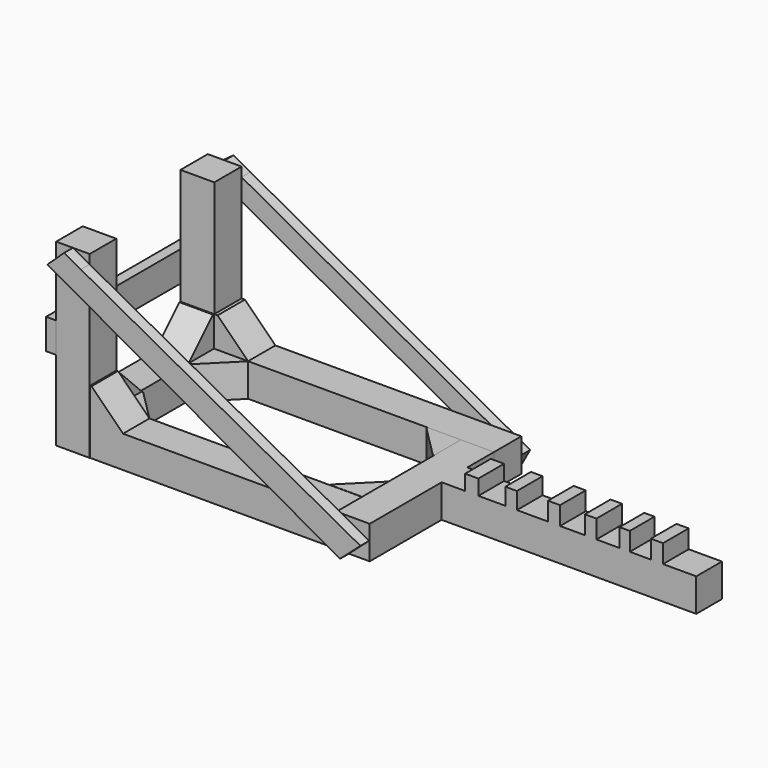
from build123d import *

# Parameters (mm, degrees)
F1_W         = 151.4005884528
F1_H         = 15.9740373492
F2_DEPTH     = 15.494
F3_W         = 151.6942754388
F3_H         = 16.5184233338
F4_DEPTH     = 16.002
F5_W         = 16.2231996655
F5_H         = 16.002
F6_DEPTH     = 75.184
F7_W         = 16.0225182772
F7_H         = 16.002
F8_DEPTH     = 75.184
F9_W         = 16.3512788713
F9_H         = 16.5184233338
F10_DEPTH    = 70.866
F11_W        = 16.2231996655
F11_H        = 16.0698437091
F12_DEPTH    = 70.866
F14_DEPTH    = 5.334
F16_DEPTH    = 5.334
F17_W        = 16.8584026396
F17_H        = 16.5184233338
F18_DEPTH    = 14.732
F19_W        = 74.9277304858
F19_H        = 14.6761201322
F19_W_2      = 16.5184233338
F20_DEPTH    = 5.08
F21_W        = 15.5249363743
F21_H        = 16.002
F22_DEPTH    = 123.19
F23_W        = 6.4162164927
F23_H        = 15.5249363743
F24_DEPTH    = 7.366
F25_W        = 5.6235641241
F25_H        = 15.5249363743
F27_DEPTH    = 8.128
F26_W        = 5.8422535658
F26_H        = 15.5089418404
F28_DEPTH    = 8.89
F29_W        = 5.5933743715
F29_H        = 15.5249363743
F31_DEPTH    = 8.89
F30_W        = 4.9718916416
F30_H        = 14.9346985854
F32_DEPTH    = 8.89
F33_W        = 5.9155483258
F33_H        = 15.5249363743
F34_DEPTH    = 8.89
F35_W        = 15.9818716347
F35_H        = 15.9740373492
F36_DEPTH    = 15.24
F37_SIZE     = 15.23999
F38_T4_DEPTH = 94.903320807
F39_W        = 16.2231996655
F39_H        = 15.4443886131
F40_DEPTH    = 14.732
F41_T4_DEPTH = 94.6080971387
F43_DEPTH    = 15.24
F44_SIZE     = 15.23999
F45_W        = 16.2231996655
F45_H        = 15.8491954207
F46_DEPTH    = 14.732
F47_T1_DEPTH = 94.6080971387
F48_W        = 15.3119927272
F48_H        = 16.002
F49_DEPTH    = 16.51
F50_SIZE     = 15.24
F51_W        = 16.0471685231
F51_H        = 16.002
F53_DEPTH    = 16.002
F52_W        = 15.7556738704
F52_H        = 15.5713185668
F54_DEPTH    = 16.002
F55_SIZE     = 15.24
F56_SIZE     = 15.24


# Not quite as in the source:
# - a fillet or chamfer that OpenCascade refuses, or shapes differently, is made with other operations: its cross-section is extruded or revolved along the edge and cut away or added
# - a fillet or chamfer is up to 0.001 mm smaller than in the source, because OpenCascade refuses the exact size


with BuildPart() as f2:
    # F1 (on face) → F2 (new body)
    with BuildSketch(Plane.XY):
        with Locations((-0.4072971642, -43.195284903)):
            Rectangle(F1_W, F1_H)
    extrude(amount=F2_DEPTH)

    # F35 (on face) → F36 (join)
    with BuildSketch(Plane.XY.offset(15.494)):
        with Locations((-51.8394764513, -43.195284903)):
            Rectangle(F35_W, F35_H)
    extrude(amount=F36_DEPTH)

    # F37 (size 15.24 in the source; OpenCascade refuses exactly that, so slightly less here)
    f37_edges = [f2.edges().sort_by_distance(p)[0] for p in [
        (-43.848541, -43.195285, 30.734),
    ]]
    chamfer(f37_edges, length=F37_SIZE)


with BuildPart() as f4:
    # F3 (on face) → F4 (new body)
    with BuildSketch(Plane.XY):
        with Locations((-0.2604536712, 32.1307359263)):
            Rectangle(F3_W, F3_H)
    extrude(amount=F4_DEPTH)

    # F9 (on face) → F10 (join)
    with BuildSketch(Plane.XY.offset(16.002)):
        with Locations((-67.931951955, 32.1307359263)):
            Rectangle(F9_W, F9_H)
    extrude(amount=F10_DEPTH)

    # F13 (on face) → F14 (join)
    with BuildSketch(Plane(origin=(0, 40.3899475932, 0), x_dir=(-1, 0, 0), z_dir=(0, 1, 0))):
        Polygon((59.7563125193, 71.958167232), (59.7563125193, 82.3752862081), (-61.0268224247, 16.002), (-42.0702156496, 16.002), align=None)
        Polygon((76.1075913906, 80.9435948159), (67.931951955, 86.868), (59.7563125193, 82.3752862081), (59.7563125193, 71.958167232), align=None)
        Polygon((-42.0702156496, 16.002), (-61.0268224247, 16.002), (-75.5866840482, 8.001), (-71.1899388967, 0), align=None)
    extrude(amount=F14_DEPTH)

    # F17 (on face) → F18 (join)
    with BuildSketch(Plane.XY.offset(16.002)):
        with Locations((-51.3271111995, 32.1307359263)):
            Rectangle(F17_W, F17_H)
    extrude(amount=F18_DEPTH)

    # F38: chamfer of 15.24 on 1 edges, made by hand


with BuildPart() as f6:
    # F5 (on face) → F6 (new body)
    with BuildSketch(Plane.XZ.offset(-23.8715242594)):
        with Locations((-67.9959915578, 8.001)):
            Rectangle(F5_W, F5_H)
    extrude(amount=F6_DEPTH)

    # F11 (on face) → F12 (join)
    with BuildSketch(Plane.XY.offset(16.002)):
        with Locations((-67.9959915578, -43.277553886)):
            Rectangle(F11_W, F11_H)
    extrude(amount=F12_DEPTH)

    # F39 (on face) → F40 (join)
    with BuildSketch(Plane.XY.offset(16.002)):
        with Locations((-67.9959915578, -27.5204377249)):
            Rectangle(F39_W, F39_H)
    extrude(amount=F40_DEPTH)

    # F41: chamfer of 15.24 on 1 edges, made by hand


with BuildPart() as f8:
    # F7 (on face) → F8 (new body)
    with BuildSketch(Plane.XZ.offset(-23.8715242594)):
        with Locations((67.5754249096, 8.001)):
            Rectangle(F7_W, F7_H)
    extrude(amount=F8_DEPTH)

    # F21 (on face) → F22 (join)
    with BuildSketch(Plane.YZ.offset(75.5866840482)):
        with Locations((-0.0333769713, 8.001)):
            Rectangle(F21_W, F21_H)
    extrude(amount=F22_DEPTH)

    # F23 (on face) → F24 (join)
    with BuildSketch(Plane.XY.offset(16.002)):
        with Locations((90.1563689113, -0.0333769713)):
            Rectangle(F23_W, F23_H)
    extrude(amount=F24_DEPTH)

    # F25 (on face) → F27 (join)
    with BuildSketch(Plane.XY.offset(16.002)):
        with Locations((109.1945394874, -0.0333769713)):
            Rectangle(F25_W, F25_H)
    extrude(amount=F27_DEPTH)

    # F26 (on face) → F28 (join)
    with BuildSketch(Plane.XY.offset(16.002)):
        with Locations((129.9700066447, -0.0413742382)):
            Rectangle(F26_W, F26_H)
    extrude(amount=F28_DEPTH)

    # F29 (on face) → F31 (join)
    with BuildSketch(Plane.XY.offset(16.002)):
        with Locations((147.6669237018, -0.0333769713)):
            Rectangle(F29_W, F29_H)
    extrude(amount=F31_DEPTH)

    # F30 (on face) → F32 (join)
    with BuildSketch(Plane.XY.offset(16.002)):
        with Locations((164.1362756491, -0.3284958657)):
            Rectangle(F30_W, F30_H)
    extrude(amount=F32_DEPTH)

    # F33 (on face) → F34 (join)
    with BuildSketch(Plane.XY.offset(16.002)):
        with Locations((179.7416785961, -0.0333769713)):
            Rectangle(F33_W, F33_H)
    extrude(amount=F34_DEPTH)

    # F52 (on face) → F54 (join)
    with BuildSketch(Plane(origin=(59.564165771, 0, 0), x_dir=(0, -1, 0), z_dir=(-1, 0, 0))):
        with Locations((27.2920625284, 7.7856592834)):
            Rectangle(F52_W, F52_H)
    extrude(amount=F54_DEPTH)

    # F56
    f56_edges = [f8.edges().sort_by_distance(p)[0] for p in [
        (43.562166, -19.414226, 7.785659),
    ]]
    chamfer(f56_edges, length=F56_SIZE)


with BuildPart() as f16:
    # F15 (on face) → F16 (new body)
    with BuildSketch(Plane.XZ.offset(51.3124757406)):
        Polygon((75.3667727113, 8.7171085179), (-59.8843917251, 82.4461491693), (-59.8843917251, 70.1829955211), (65.5179917812, 0), align=None)
        Polygon((-59.8843917251, 82.4461491693), (-67.9959915578, 86.868), (-76.1075913906, 79.2625099421), (-59.8843917251, 70.1829955211), align=None)
    extrude(amount=F16_DEPTH)


with BuildPart() as f20:
    # F19 (on face) → F20 (new body)
    with BuildSketch(Plane(origin=(-76.1075913906, 0, 0), x_dir=(0, -1, 0), z_dir=(-1, 0, 0))):
        with Locations((13.5923409835, 45.7748640329)):
            Rectangle(F19_W, F19_H)
        with Locations((-32.1307359263, 45.7748640329)):
            Rectangle(F19_W_2, F19_H)
    extrude(amount=F20_DEPTH)


with BuildPart() as f38_tool2:
    # F38_s3 → F38_t4 (new body)
    with BuildSketch(Plane.XZ.offset(15.3209244772)):
        Polygon((-42.8979098797, 15.494), (-58.1379098797, 30.734), (-42.8979098797, 30.734), align=None)
    extrude(amount=-F38_T4_DEPTH)

    split(bisect_by=Plane.XY.offset(16.002), keep=Keep.TOP)


with BuildPart() as f4_1:
    add(f4.part)

    # F38_t1: cut F38_tool2
    add(f38_tool2.part, mode=Mode.SUBTRACT)


with BuildPart() as f41_tool2:
    # F41_s3 → F41_t4 (new body)
    with BuildSketch(Plane.YZ.offset(-20.6919429885)):
        Polygon((-19.7982434183, 15.494), (-35.0382434183, 30.734), (-19.7982434183, 30.734), align=None)
    extrude(amount=-F41_T4_DEPTH)

    split(bisect_by=Plane.XY.offset(16.002), keep=Keep.TOP)


with BuildPart() as f6_1:
    add(f6.part)

    # F41_t1: cut F41_tool2
    add(f41_tool2.part, mode=Mode.SUBTRACT)


with BuildPart() as f43:
    # F42 (on face) → F43 (new body)
    with BuildSketch(Plane(origin=(0, -35.2082662284, 0), x_dir=(-1, 0, 0), z_dir=(0, 1, 0))):
        Polygon((43.8485406339, 0), (60.0956752896, 0), (60.0956752896, 15.494), (59.8304122686, 15.494), (43.8485406339, 15.494), align=None)
    extrude(amount=F43_DEPTH)

    # F44 (size 15.24 in the source; OpenCascade refuses exactly that, so slightly less here)
    f44_edges = [f43.edges().sort_by_distance(p)[0] for p in [
        (-43.848541, -19.968266, 7.747),
    ]]
    chamfer(f44_edges, length=F44_SIZE)


with BuildPart() as f46:
    # F45 (on face) → F46 (new body)
    with BuildSketch(Plane.XY.offset(16.002)):
        with Locations((-67.9959915578, 15.9469265491)):
            Rectangle(F45_W, F45_H)
    extrude(amount=F46_DEPTH)

    # F47: chamfer of 15.24 on 1 edges, made by hand

    # F47_s2 → F47_t1 (cut)
    with BuildSketch(Plane.YZ.offset(-115.3000401272)):
        Polygon((8.0223288387, 15.494), (23.2623288387, 30.734), (8.0223288387, 30.734), align=None)
    extrude(amount=F47_T1_DEPTH, mode=Mode.SUBTRACT)


with BuildPart() as f49:
    # F48 (on face) → F49 (new body)
    with BuildSketch(Plane.YZ.offset(-59.8843917251)):
        with Locations((16.2155278958, 8.001)):
            Rectangle(F48_W, F48_H)
    extrude(amount=F49_DEPTH)

    # F50
    f50_edges = [f49.edges().sort_by_distance(p)[0] for p in [
        (-43.374392, 8.559532, 8.001),
    ]]
    chamfer(f50_edges, length=F50_SIZE)


with BuildPart() as f53:
    # F51 (on face) → F53 (new body)
    with BuildSketch(Plane(origin=(59.564165771, 0, 0), x_dir=(0, -1, 0), z_dir=(-1, 0, 0))):
        with Locations((-15.8479399979, 8.001)):
            Rectangle(F51_W, F51_H)
    extrude(amount=F53_DEPTH)

    # F55
    f55_edges = [f53.edges().sort_by_distance(p)[0] for p in [
        (43.562166, 7.824356, 8.001),
    ]]
    chamfer(f55_edges, length=F55_SIZE)


solid = Compound([f2.part, f8.part, f16.part, f20.part, f4_1.part, f6_1.part, f43.part, f46.part, f49.part, f53.part])
